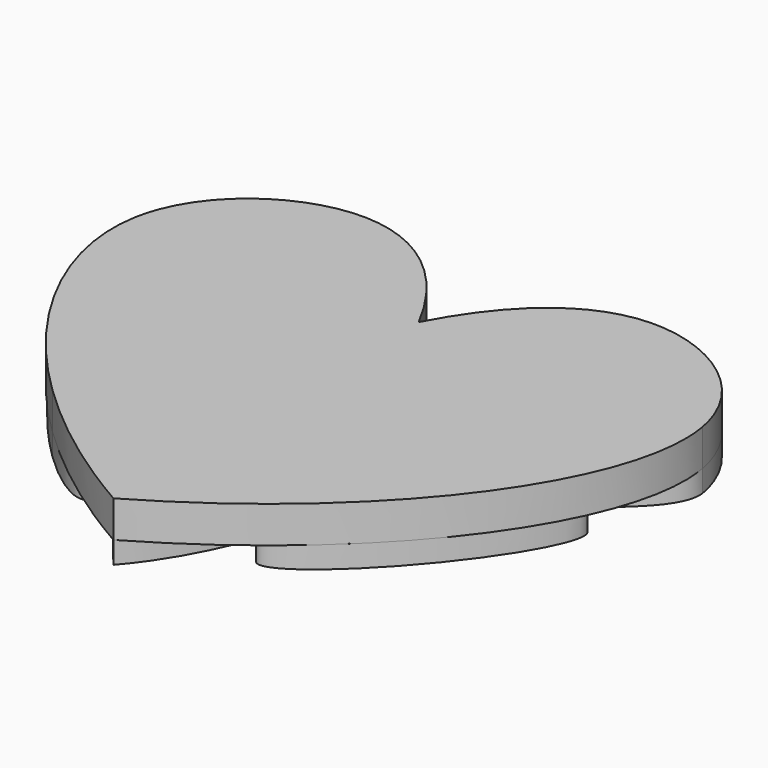
from build123d import *

# Parameters (mm, degrees)
F1_DEPTH = 5
F2_DEPTH = 3
F3_DEPTH = 5


# Not quite as in the source:
# - a feature names something its author has since deleted; it is built from what else it names


with BuildPart() as f1:
    # F0 (on Top) → F1 (new body)
    with BuildSketch(Plane.XY):
        with BuildLine():
            add(Edge.make_bspline(
                [(0, 0), (5.8826601211, 11.2702567006), (20.8111578849, 20.6386629418), (37.2014190882, 8.6220207342), (38.749657821, 0)],
                knots=[0, 0, 0, 0, 0.2865659188, 0.5520449891, 0.5520449891, 0.5520449891, 0.5520449891], degree=3))
            add(Edge.make_bspline(
                [(0, 0), (-5.8826601211, 11.2702567006), (-20.8111578849, 20.6386629418), (-37.2014190882, 8.6220207342), (-38.749657821, 0)],
                knots=[0, 0, 0, 0, 0.2865659188, 0.5520449891, 0.5520449891, 0.5520449891, 0.5520449891], degree=3))
            add(Edge.make_bspline(
                [(-38.749657821, 0), (-39.4012299945, -6.6213969341), (-9.0327868439, -20.6953577001), (-8.685916815, -42.126413839), (0, -52.1089205623)],
                knots=[0, 0, 0, 0, 0.4867027196, 1, 1, 1, 1], degree=3))
            add(Edge.make_bspline(
                [(38.749657821, 0), (39.4012299945, -6.6213969341), (9.0327868439, -20.6953577001), (8.685916815, -42.126413839), (0, -52.1089205623)],
                knots=[0, 0, 0, 0, 0.4867027196, 1, 1, 1, 1], degree=3))
        make_face()
        with BuildLine():
            add(Edge.make_bspline(
                [(0, 0), (-8.039671318, 3.887850868), (-21.0375310132, 10.3979423013), (-34.1851204628, -0.0331959557), (-22.9358554941, -11.1083712256), (-9.0780722669, -20.9680892381), (-4.1014407761, -34.0341217816), (0, -39.8491583765)],
                knots=[0, 0, 0, 0, 0.236574756, 0.3977476477, 0.5702206455, 0.7762521683, 1, 1, 1, 1], degree=3))
            add(Edge.make_bspline(
                [(0, 0), (8.039671318, 3.887850868), (21.0375310132, 10.3979423013), (34.1851204628, -0.0331959557), (22.9358554941, -11.1083712256), (9.0780722669, -20.9680892381), (4.1014407761, -34.0341217816), (0, -39.8491583765)],
                knots=[0, 0, 0, 0, 0.236574756, 0.3977476477, 0.5702206455, 0.7762521683, 1, 1, 1, 1], degree=3))
        make_face(mode=Mode.SUBTRACT)
        with BuildLine():
            add(Edge.make_bspline(
                [(0, 0), (8.039671318, 3.887850868), (21.0375310132, 10.3979423013), (34.1851204628, -0.0331959557), (22.9358554941, -11.1083712256), (9.0780722669, -20.9680892381), (4.1014407761, -34.0341217816), (0, -39.8491583765)],
                knots=[0, 0, 0, 0, 0.236574756, 0.3977476477, 0.5702206455, 0.7762521683, 1, 1, 1, 1], degree=3))
            add(Edge.make_bspline(
                [(0, 0), (-8.039671318, 3.887850868), (-21.0375310132, 10.3979423013), (-34.1851204628, -0.0331959557), (-22.9358554941, -11.1083712256), (-9.0780722669, -20.9680892381), (-4.1014407761, -34.0341217816), (0, -39.8491583765)],
                knots=[0, 0, 0, 0, 0.236574756, 0.3977476477, 0.5702206455, 0.7762521683, 1, 1, 1, 1], degree=3))
        make_face()
        with BuildLine():
            add(Edge.make_bspline(
                [(0, -4.2843823321), (-4.3131672708, -0.5965221259), (-13.217639527, 3.3797390078), (-19.1463981552, -11.3037035401), (-7.8477509016, -17.6284155745), (0, -23.0948515236)],
                knots=[0, 0, 0, 0, 0.3199063089, 0.5905308347, 1, 1, 1, 1], degree=3))
            add(Edge.make_bspline(
                [(0, -4.2843823321), (4.3131672708, -0.5965221259), (13.217639527, 3.3797390078), (19.1463981552, -11.3037035401), (7.8477509016, -17.6284155745), (0, -23.0948515236)],
                knots=[0, 0, 0, 0, 0.3199063089, 0.5905308347, 1, 1, 1, 1], degree=3))
        make_face(mode=Mode.SUBTRACT)
        with BuildLine():
            add(Edge.make_bspline(
                [(0, -4.2843823321), (4.3131672708, -0.5965221259), (13.217639527, 3.3797390078), (19.1463981552, -11.3037035401), (7.8477509016, -17.6284155745), (0, -23.0948515236)],
                knots=[0, 0, 0, 0, 0.3199063089, 0.5905308347, 1, 1, 1, 1], degree=3))
            add(Edge.make_bspline(
                [(0, -4.2843823321), (-4.3131672708, -0.5965221259), (-13.217639527, 3.3797390078), (-19.1463981552, -11.3037035401), (-7.8477509016, -17.6284155745), (0, -23.0948515236)],
                knots=[0, 0, 0, 0, 0.3199063089, 0.5905308347, 1, 1, 1, 1], degree=3))
        make_face()
        with BuildLine():
            add(Edge.make_bspline(
                [(-38.749657821, 0), (-39.4012299945, -6.6213969341), (-9.0327868439, -20.6953577001), (-8.685916815, -42.126413839), (0, -52.1089205623)],
                knots=[0, 0, 0, 0, 0.4867027196, 1, 1, 1, 1], degree=3))
            add(Edge.make_bspline(
                [(-38.749657821, 0), (-40.5608709324, -10.0865045363), (-33.7038328837, -24.0640985889), (-20.6823740602, -36.6602716931)],
                knots=[0.5520449891, 0.5520449891, 0.5520449891, 0.5520449891, 0.8626167135, 0.8626167135, 0.8626167135, 0.8626167135], degree=3))
            add(Edge.make_bspline(
                [(-20.6823740602, -36.6602716931), (-14.9222527489, -42.2322652862), (-7.9558844229, -47.5339439616), (0, -52.1089205623)],
                knots=[0.8626167135, 0.8626167135, 0.8626167135, 0.8626167135, 1, 1, 1, 1], degree=3))
        make_face()
        with BuildLine():
            add(Edge.make_bspline(
                [(-20.6823740602, -36.6602716931), (-13.3891185223, -43.7153269099), (-11.5241668889, -42.155893369)],
                knots=[5.1678619688, 5.1678619688, 5.1678619688, 6.2831853072, 6.2831853072, 6.2831853072], degree=2, weights=[1, 0.8484948826, 1]))
            add(Edge.make_bspline(
                [(-11.5241668889, -42.155893369), (-1.0796225414, -33.4223838863), (-31.3037078069, -15.2856312429), (-61.5277930724, 2.8511214004), (-20.6823740602, -36.6602716931)],
                knots=[0, 0, 0, 2.5839309844, 2.5839309844, 5.1678619688, 5.1678619688, 5.1678619688], degree=2, weights=[1, 0.2752318272, 1, 0.2752318272, 1]))
        make_face(mode=Mode.SUBTRACT)
        with BuildLine():
            add(Edge.make_bspline(
                [(38.749657821, 0), (40.5608709326, -10.0865045375), (33.7038328821, -24.0640985922), (20.6823740557, -36.6602716974)],
                knots=[0.5520449891, 0.5520449891, 0.5520449891, 0.5520449891, 0.8626167135, 0.8626167135, 0.8626167135, 0.8626167135], degree=3))
            add(Edge.make_bspline(
                [(38.749657821, 0), (39.4012299945, -6.6213969341), (9.0327868439, -20.6953577001), (8.685916815, -42.126413839), (0, -52.1089205623)],
                knots=[0, 0, 0, 0, 0.4867027196, 1, 1, 1, 1], degree=3))
            add(Edge.make_bspline(
                [(20.6823740557, -36.6602716974), (14.9222527452, -42.232265289), (7.9558844208, -47.5339439628), (0, -52.1089205623)],
                knots=[0.8626167135, 0.8626167135, 0.8626167135, 0.8626167135, 1, 1, 1, 1], degree=3))
        make_face()
        with BuildLine():
            add(Edge.make_bspline(
                [(20.6823740557, -36.6602716974), (61.5277930795, 2.8511213993), (31.3037078086, -15.2856312419), (1.0796225376, -33.4223838832), (11.5241668889, -42.155893369)],
                knots=[1.115323338, 1.115323338, 1.115323338, 3.6992543226, 3.6992543226, 6.2831853072, 6.2831853072, 6.2831853072], degree=2, weights=[1, 0.2752318271, 1, 0.2752318271, 1]))
            add(Edge.make_bspline(
                [(11.5241668889, -42.155893369), (13.3891185215, -43.7153269093), (20.6823740557, -36.6602716974)],
                knots=[0, 0, 0, 1.115323338, 1.115323338, 1.115323338], degree=2, weights=[1, 0.8484948827, 1]))
        make_face(mode=Mode.SUBTRACT)
        with BuildLine():
            add(Edge.make_bspline(
                [(-11.5241668889, -42.155893369), (-1.0796225414, -33.4223838863), (-31.3037078069, -15.2856312429), (-61.5277930724, 2.8511214004), (-20.6823740602, -36.6602716931)],
                knots=[0, 0, 0, 2.5839309844, 2.5839309844, 5.1678619688, 5.1678619688, 5.1678619688], degree=2, weights=[1, 0.2752318272, 1, 0.2752318272, 1]))
            add(Edge.make_bspline(
                [(-20.6823740602, -36.6602716931), (-13.3891185223, -43.7153269099), (-11.5241668889, -42.155893369)],
                knots=[5.1678619688, 5.1678619688, 5.1678619688, 6.2831853072, 6.2831853072, 6.2831853072], degree=2, weights=[1, 0.8484948826, 1]))
        make_face()
        with BuildLine():
            add(Edge.make_bspline(
                [(11.5241668889, -42.155893369), (13.3891185215, -43.7153269093), (20.6823740557, -36.6602716974)],
                knots=[0, 0, 0, 1.115323338, 1.115323338, 1.115323338], degree=2, weights=[1, 0.8484948827, 1]))
            add(Edge.make_bspline(
                [(20.6823740557, -36.6602716974), (61.5277930795, 2.8511213993), (31.3037078086, -15.2856312419), (1.0796225376, -33.4223838832), (11.5241668889, -42.155893369)],
                knots=[1.115323338, 1.115323338, 1.115323338, 3.6992543226, 3.6992543226, 6.2831853072, 6.2831853072, 6.2831853072], degree=2, weights=[1, 0.2752318271, 1, 0.2752318271, 1]))
        make_face()
    extrude(amount=F1_DEPTH)

    # F0 (on Top) → F2 (join)
    with BuildSketch(Plane.XY):
        with BuildLine():
            add(Edge.make_bspline(
                [(0, 0), (5.8826601211, 11.2702567006), (20.8111578849, 20.6386629418), (37.2014190882, 8.6220207342), (38.749657821, 0)],
                knots=[0, 0, 0, 0, 0.2865659188, 0.5520449891, 0.5520449891, 0.5520449891, 0.5520449891], degree=3))
            add(Edge.make_bspline(
                [(0, 0), (-5.8826601211, 11.2702567006), (-20.8111578849, 20.6386629418), (-37.2014190882, 8.6220207342), (-38.749657821, 0)],
                knots=[0, 0, 0, 0, 0.2865659188, 0.5520449891, 0.5520449891, 0.5520449891, 0.5520449891], degree=3))
            add(Edge.make_bspline(
                [(-38.749657821, 0), (-39.4012299945, -6.6213969341), (-9.0327868439, -20.6953577001), (-8.685916815, -42.126413839), (0, -52.1089205623)],
                knots=[0, 0, 0, 0, 0.4867027196, 1, 1, 1, 1], degree=3))
            add(Edge.make_bspline(
                [(38.749657821, 0), (39.4012299945, -6.6213969341), (9.0327868439, -20.6953577001), (8.685916815, -42.126413839), (0, -52.1089205623)],
                knots=[0, 0, 0, 0, 0.4867027196, 1, 1, 1, 1], degree=3))
        make_face()
        with BuildLine():
            add(Edge.make_bspline(
                [(0, 0), (-8.039671318, 3.887850868), (-21.0375310132, 10.3979423013), (-34.1851204628, -0.0331959557), (-22.9358554941, -11.1083712256), (-9.0780722669, -20.9680892381), (-4.1014407761, -34.0341217816), (0, -39.8491583765)],
                knots=[0, 0, 0, 0, 0.236574756, 0.3977476477, 0.5702206455, 0.7762521683, 1, 1, 1, 1], degree=3))
            add(Edge.make_bspline(
                [(0, 0), (8.039671318, 3.887850868), (21.0375310132, 10.3979423013), (34.1851204628, -0.0331959557), (22.9358554941, -11.1083712256), (9.0780722669, -20.9680892381), (4.1014407761, -34.0341217816), (0, -39.8491583765)],
                knots=[0, 0, 0, 0, 0.236574756, 0.3977476477, 0.5702206455, 0.7762521683, 1, 1, 1, 1], degree=3))
        make_face(mode=Mode.SUBTRACT)
        with BuildLine():
            add(Edge.make_bspline(
                [(0, 0), (8.039671318, 3.887850868), (21.0375310132, 10.3979423013), (34.1851204628, -0.0331959557), (22.9358554941, -11.1083712256), (9.0780722669, -20.9680892381), (4.1014407761, -34.0341217816), (0, -39.8491583765)],
                knots=[0, 0, 0, 0, 0.236574756, 0.3977476477, 0.5702206455, 0.7762521683, 1, 1, 1, 1], degree=3))
            add(Edge.make_bspline(
                [(0, 0), (-8.039671318, 3.887850868), (-21.0375310132, 10.3979423013), (-34.1851204628, -0.0331959557), (-22.9358554941, -11.1083712256), (-9.0780722669, -20.9680892381), (-4.1014407761, -34.0341217816), (0, -39.8491583765)],
                knots=[0, 0, 0, 0, 0.236574756, 0.3977476477, 0.5702206455, 0.7762521683, 1, 1, 1, 1], degree=3))
        make_face()
        with BuildLine():
            add(Edge.make_bspline(
                [(0, -4.2843823321), (-4.3131672708, -0.5965221259), (-13.217639527, 3.3797390078), (-19.1463981552, -11.3037035401), (-7.8477509016, -17.6284155745), (0, -23.0948515236)],
                knots=[0, 0, 0, 0, 0.3199063089, 0.5905308347, 1, 1, 1, 1], degree=3))
            add(Edge.make_bspline(
                [(0, -4.2843823321), (4.3131672708, -0.5965221259), (13.217639527, 3.3797390078), (19.1463981552, -11.3037035401), (7.8477509016, -17.6284155745), (0, -23.0948515236)],
                knots=[0, 0, 0, 0, 0.3199063089, 0.5905308347, 1, 1, 1, 1], degree=3))
        make_face(mode=Mode.SUBTRACT)
        with BuildLine():
            add(Edge.make_bspline(
                [(0, -4.2843823321), (4.3131672708, -0.5965221259), (13.217639527, 3.3797390078), (19.1463981552, -11.3037035401), (7.8477509016, -17.6284155745), (0, -23.0948515236)],
                knots=[0, 0, 0, 0, 0.3199063089, 0.5905308347, 1, 1, 1, 1], degree=3))
            add(Edge.make_bspline(
                [(0, -4.2843823321), (-4.3131672708, -0.5965221259), (-13.217639527, 3.3797390078), (-19.1463981552, -11.3037035401), (-7.8477509016, -17.6284155745), (0, -23.0948515236)],
                knots=[0, 0, 0, 0, 0.3199063089, 0.5905308347, 1, 1, 1, 1], degree=3))
        make_face()
    extrude(amount=-F2_DEPTH)

    # F0 (on Top) → F3 (join)
    with BuildSketch(Plane.XY):
        with BuildLine():
            add(Edge.make_bspline(
                [(0, 0), (8.039671318, 3.887850868), (21.0375310132, 10.3979423013), (34.1851204628, -0.0331959557), (22.9358554941, -11.1083712256), (9.0780722669, -20.9680892381), (4.1014407761, -34.0341217816), (0, -39.8491583765)],
                knots=[0, 0, 0, 0, 0.236574756, 0.3977476477, 0.5702206455, 0.7762521683, 1, 1, 1, 1], degree=3))
            add(Edge.make_bspline(
                [(0, 0), (-8.039671318, 3.887850868), (-21.0375310132, 10.3979423013), (-34.1851204628, -0.0331959557), (-22.9358554941, -11.1083712256), (-9.0780722669, -20.9680892381), (-4.1014407761, -34.0341217816), (0, -39.8491583765)],
                knots=[0, 0, 0, 0, 0.236574756, 0.3977476477, 0.5702206455, 0.7762521683, 1, 1, 1, 1], degree=3))
        make_face()
        with BuildLine():
            add(Edge.make_bspline(
                [(0, -4.2843823321), (-4.3131672708, -0.5965221259), (-13.217639527, 3.3797390078), (-19.1463981552, -11.3037035401), (-7.8477509016, -17.6284155745), (0, -23.0948515236)],
                knots=[0, 0, 0, 0, 0.3199063089, 0.5905308347, 1, 1, 1, 1], degree=3))
            add(Edge.make_bspline(
                [(0, -4.2843823321), (4.3131672708, -0.5965221259), (13.217639527, 3.3797390078), (19.1463981552, -11.3037035401), (7.8477509016, -17.6284155745), (0, -23.0948515236)],
                knots=[0, 0, 0, 0, 0.3199063089, 0.5905308347, 1, 1, 1, 1], degree=3))
        make_face(mode=Mode.SUBTRACT)
    extrude(amount=-F3_DEPTH)


with BuildPart() as f2:
    # F0 (on Top) → F2, piece 2 (new body)
    with BuildSketch(Plane.XY):
        with BuildLine():
            add(Edge.make_bspline(
                [(11.5241668889, -42.155893369), (13.3891185215, -43.7153269093), (20.6823740557, -36.6602716974)],
                knots=[0, 0, 0, 1.115323338, 1.115323338, 1.115323338], degree=2, weights=[1, 0.8484948827, 1]))
            add(Edge.make_bspline(
                [(20.6823740557, -36.6602716974), (61.5277930795, 2.8511213993), (31.3037078086, -15.2856312419), (1.0796225376, -33.4223838832), (11.5241668889, -42.155893369)],
                knots=[1.115323338, 1.115323338, 1.115323338, 3.6992543226, 3.6992543226, 6.2831853072, 6.2831853072, 6.2831853072], degree=2, weights=[1, 0.2752318271, 1, 0.2752318271, 1]))
        make_face()
    extrude(amount=-F2_DEPTH)


with BuildPart() as f2b:
    # F0 (on Top) → F2, piece 3 (new body)
    with BuildSketch(Plane.XY):
        with BuildLine():
            add(Edge.make_bspline(
                [(-11.5241668889, -42.155893369), (-1.0796225414, -33.4223838863), (-31.3037078069, -15.2856312429), (-61.5277930724, 2.8511214004), (-20.6823740602, -36.6602716931)],
                knots=[0, 0, 0, 2.5839309844, 2.5839309844, 5.1678619688, 5.1678619688, 5.1678619688], degree=2, weights=[1, 0.2752318272, 1, 0.2752318272, 1]))
            add(Edge.make_bspline(
                [(-20.6823740602, -36.6602716931), (-13.3891185223, -43.7153269099), (-11.5241668889, -42.155893369)],
                knots=[5.1678619688, 5.1678619688, 5.1678619688, 6.2831853072, 6.2831853072, 6.2831853072], degree=2, weights=[1, 0.8484948826, 1]))
        make_face()
    extrude(amount=-F2_DEPTH)


solid = Compound([f1.part, f2.part, f2b.part])
